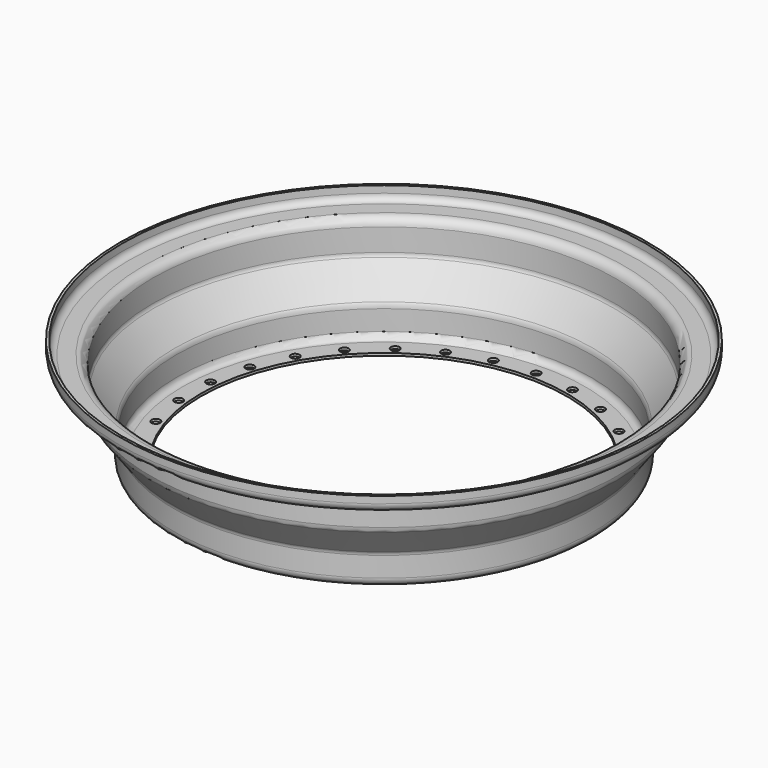
from build123d import *

# Parameters (mm, degrees)
F2_R            = 3.5
F3_DEPTH        = 2.001
F3_COPIES_COUNT = 30


# Not quite as in the source:
# - a pattern or mirror of a feature is missing from the dataset's text; its kind, count and spacing are read off the source's solid


with BuildPart() as f1:
    # F0 (on Front) → F1 (revolve)
    with BuildSketch(Plane.XZ):
        with BuildLine():
            Line((-164, 0), (-149, 0))
            Line((-149, 0), (-149, 2))
            Line((-149, 2), (-164, 2))
            ThreePointArc((-164, 2), (-167.5355339059, 3.4644660941), (-169, 7))
            Line((-169, 7), (-169, 23.3435332173))
            ThreePointArc((-169, 23.3435332173), (-169.3551615249, 25.5449240594), (-170.3846061827, 27.5229293791))
            Line((-170.3846061827, 27.5229293791), (-187.5109955838, 50.5337705231))
            ThreePointArc((-187.5109955838, 50.5337705231), (-188.2463131965, 51.9466314657), (-188.5, 53.5190534957))
            Line((-188.5, 53.5190534957), (-188.5, 71.8625867131))
            ThreePointArc((-188.5, 71.8625867131), (-190.8895043975, 76.5028494379), (-195.8252362977, 78.2))
            Line((-195.8252362977, 78.2), (-207.9317760463, 78.2))
            ThreePointArc((-207.9317760463, 78.2), (-211.4673099522, 79.6644660941), (-212.9317760463, 83.2))
            Line((-212.9317760463, 83.2), (-212.9317760463, 88.9))
            Line((-212.9317760463, 88.9), (-214.9317760463, 88.9))
            Line((-214.9317760463, 88.9), (-214.9317760463, 83.2))
            ThreePointArc((-214.9317760463, 83.2), (-212.8815235146, 78.2502525317), (-207.9317760463, 76.2))
            Line((-207.9317760463, 76.2), (-195.5, 76.2))
            ThreePointArc((-195.5, 76.2), (-191.9644660941, 74.7355339059), (-190.5, 71.2))
            Line((-190.5, 71.2), (-190.5, 53.5190534957))
            ThreePointArc((-190.5, 53.5190534957), (-190.1448384751, 51.3176626537), (-189.1153938173, 49.339657334))
            Line((-189.1153938173, 49.339657334), (-171.9890044162, 26.32881619))
            ThreePointArc((-171.9890044162, 26.32881619), (-171.2536868035, 24.9159552474), (-171, 23.3435332173))
            Line((-171, 23.3435332173), (-171, 7))
            ThreePointArc((-171, 7), (-168.9497474683, 2.0502525317), (-164, 0))
        make_face()
    revolve(axis=Axis((0, 0, 22.5889328867), (0, 0, 1)))

    # F2 (on face) → F3 (cut, through all)
    with BuildSketch(Plane.XY.offset(2)):
        with Locations((0, 155)):
            Circle(F2_R)
    f3 = extrude(amount=-F3_DEPTH, mode=Mode.SUBTRACT)

    # F3_copies: F3 ×30 about axis
    f3_copies_axis = Axis((0, 0, 0), (0, 0, 1))
    for i in range(1, F3_COPIES_COUNT):
        add(f3.rotate(f3_copies_axis, i * 360 / F3_COPIES_COUNT), mode=Mode.SUBTRACT)


solid = f1.part
